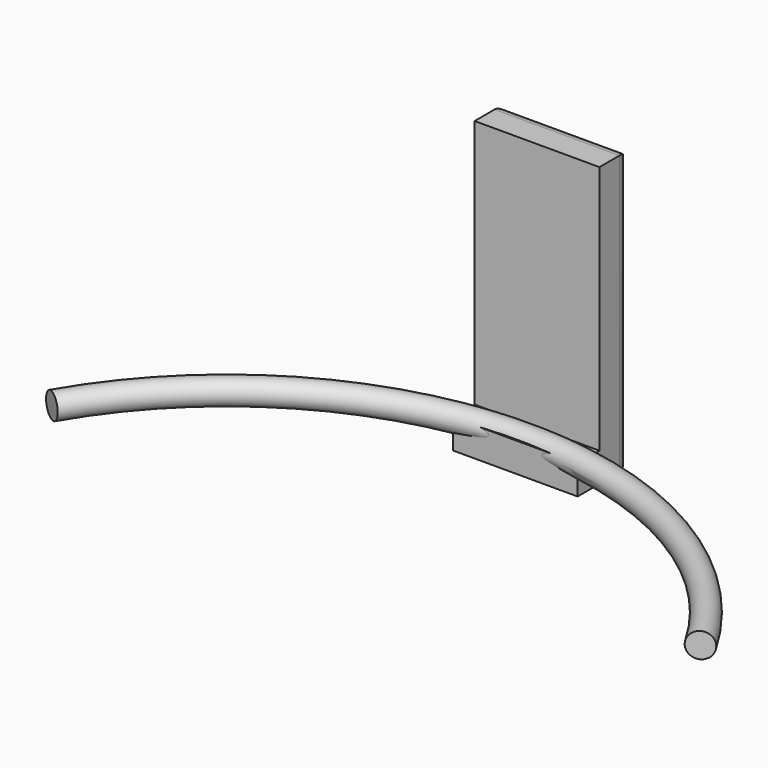
from build123d import *

# Parameters (mm, degrees)
F0_R          = 5
F1_ANGLE_BACK = 60
F1_ANGLE      = 120
F2_W          = 25.9252840082
F2_H          = 11.7293265872
F3_DEPTH      = 25
F3_DEPTH_BACK = 25
F4_W          = 50
F4_H          = 15
F5_DEPTH      = 100
F6_R          = 5


# Not quite as in the source:
# - a feature of the source that left no trace in its solid (it failed there, or was rolled back) is left out


with BuildPart() as f1:
    # F0 (on Right) → F1 (revolve)
    with BuildSketch(Plane.YZ, mode=Mode.PRIVATE) as f1_sk:
        with Locations((30.3885055535, 0)):
            Circle(F0_R)
    revolve(f1_sk.sketch.rotate(Axis((0, -119.6114944465, -16.3725827584), (0, 0, -1)), -F1_ANGLE_BACK), axis=Axis((0, -119.6114944465, -16.3725827584), (0, 0, -1)), revolution_arc=F1_ANGLE)

    # F2 (on Right) → F3 (join, two sides)
    with BuildSketch(Plane.YZ) as f3_sk:
        with Locations((37.9626420041, -4.1353367064)):
            Rectangle(F2_W, F2_H)
    extrude(amount=F3_DEPTH)
    extrude(f3_sk.sketch, amount=-F3_DEPTH_BACK)

    # F4 (on face) → F5 (join)
    with BuildSketch(Plane.XY.offset(1.7293265872)):
        with Locations((0, 43.4252840082)):
            Rectangle(F4_W, F4_H)
    extrude(amount=F5_DEPTH)

    # F6
    f6_edges = [f1.edges().sort_by_distance(p)[0] for p in [
        (0, 50.925284, -10),
        (25, 50.925284, 45.864663),
        (0, 50.925284, 101.729327),
        (-25, 50.925284, 45.864663),
    ]]
    fillet(f6_edges, radius=F6_R)


solid = f1.part
